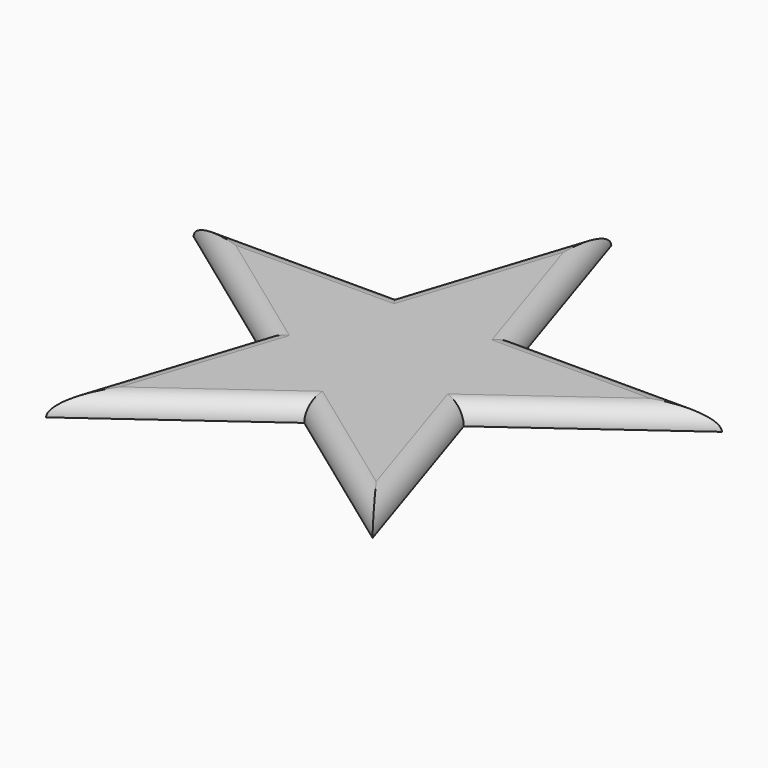
from build123d import *

# Parameters (mm, degrees)
F1_DEPTH = 2.5
F2_R     = 2.49999


# Not quite as in the source:
# - a fillet or chamfer is up to 0.001 mm smaller than in the source, because OpenCascade refuses the exact size


with BuildPart() as f1:
    # F0 (on Top) → F1 (new body)
    with BuildSketch(Plane.XY):
        Polygon((-8.4192745609, 11.5881372891), (-35.6646193611, 11.5881372891), (-13.6226724001, -4.4262745781), (-22.041946961, -30.3381372891), (0, -14.3237254219), (22.041946961, -30.3381372891), (13.6226724001, -4.4262745781), (35.6646193611, 11.5881372891), (8.4192745609, 11.5881372891), (0, 37.5), align=None)
    extrude(amount=F1_DEPTH)

    # F2 (radius 2.5 in the source; OpenCascade refuses exactly that, so slightly less here)
    f2_edges = [f1.edges().sort_by_distance(p)[0] for p in [
        (-4.209637, 24.544069, 2.5),
        (-22.041947, 11.588137, 2.5),
        (-24.643646, 3.580931, 2.5),
        (-17.83231, -17.382206, 2.5),
        (11.020973, -22.330931, 2.5),
        (17.83231, -17.382206, 2.5),
        (24.643646, 3.580931, 2.5),
        (22.041947, 11.588137, 2.5),
        (4.209637, 24.544069, 2.5),
        (-11.020973, -22.330931, 2.5),
    ]]
    fillet(f2_edges, radius=F2_R)


solid = f1.part
